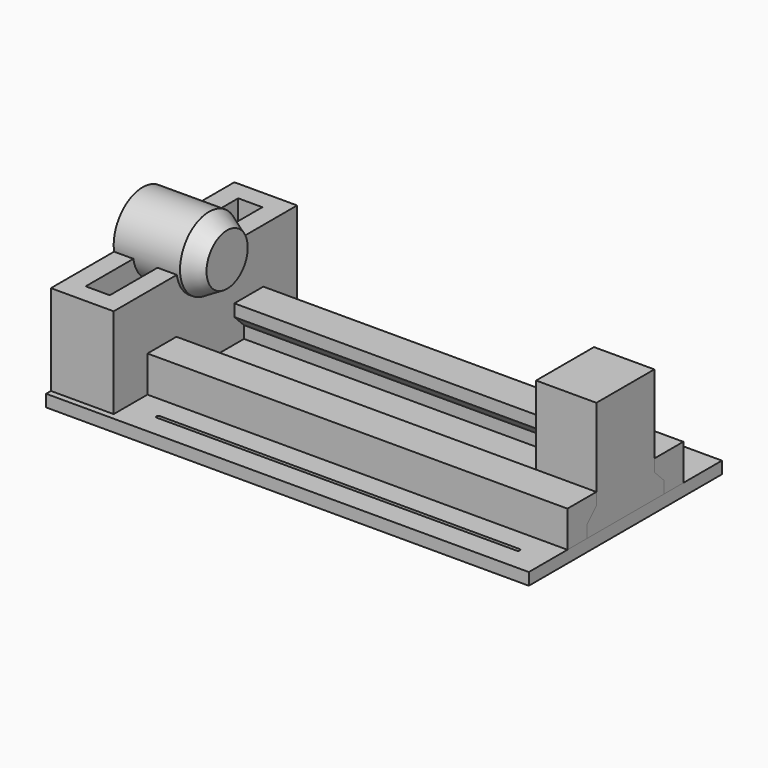
from build123d import *

# Parameters (mm, degrees)
F0_W      = 800
F0_H      = 400
F1_DEPTH  = 20
F2_W      = 40
F2_H      = 32
F3_DEPTH  = 150
F5_DEPTH  = 800.001
F6_R      = 60
F7_DEPTH  = 110
F8_R      = 60
F9_DEPTH  = 30
F9_TAPER  = 30
F11_DEPTH = 696
F14_DEPTH = 100
F17_DEPTH = 20.001


# Not quite as in the source:
# - a pattern or mirror of a feature is missing from the dataset's text; its kind, count and spacing are read off the source's solid


with BuildPart() as f1:
    # F0 (on Top) → F1 (new body)
    with BuildSketch(Plane.XY):
        Rectangle(F0_W, F0_H)
    extrude(amount=F1_DEPTH)

    # F16 (on face) → F17 (cut, through all)
    with BuildSketch(Plane.XY.offset(20)):
        with BuildLine():
            ThreePointArc((-246, -157), (-249, -160), (-246, -163))
            Line((-246, -163), (350, -163))
            ThreePointArc((350, -163), (353, -160), (350, -157))
            Line((350, -157), (-246, -157))
        make_face()
    f17 = extrude(amount=-F17_DEPTH, mode=Mode.SUBTRACT)

    # F17_copies: F17 across plane
    add(f17.mirror(Plane.ZX), mode=Mode.SUBTRACT)


with BuildPart() as f3:
    # F2 (on face) → F3 (new body)
    with BuildSketch(Plane.XY.offset(20)):
        Polygon((-400, 190), (-400, -190), (-368, -190), (-368, -158), (-368, 158), (-368, 190), align=None)
        Polygon((-328, -158), (-328, -190), (-296, -190), (-296, 190), (-328, 190), (-328, 158), align=None)
        with Locations((-348, -174)):
            Rectangle(F2_W, F2_H)
        with Locations((-348, 174)):
            Rectangle(F2_W, F2_H)
    extrude(amount=F3_DEPTH)

    # F4 (on face) → F5 (cut, through all)
    with BuildSketch(Plane(origin=(-400, 0, 0), x_dir=(0, -1, 0), z_dir=(-1, 0, 0))):
        with BuildLine():
            ThreePointArc((59.160797831, 170), (59.7898313673, 174.9824243832), (60, 180))
            ThreePointArc((60, 180), (-5.0175756168, 239.7898313673), (-59.160797831, 170))
            Line((-59.160797831, 170), (59.160797831, 170))
        make_face()
        with BuildLine():
            Line((59.160797831, 170), (-59.160797831, 170))
            ThreePointArc((-59.160797831, 170), (0, 120), (59.160797831, 170))
        make_face()
    extrude(amount=-F5_DEPTH, mode=Mode.SUBTRACT)


with BuildPart() as f7:
    # F6 (on face) → F7 (new body)
    with BuildSketch(Plane(origin=(-400, 0, 0), x_dir=(0, -1, 0), z_dir=(-1, 0, 0))):
        with Locations((0, 180)):
            Circle(F6_R)
    extrude(amount=-F7_DEPTH)

    # F8 (on face) → F9 (join)
    with BuildSketch(Plane.YZ.offset(-290)):
        with Locations((0, 180)):
            Circle(F8_R)
    extrude(amount=F9_DEPTH, taper=F9_TAPER)


with BuildPart() as f11:
    # F10 (on face) → F11 (new body, through all)
    with BuildSketch(Plane.YZ.offset(-296)):
        Polygon((-120, 20), (-80, 20), (-80, 40), (-60, 60), (-60, 80), (-120, 80), align=None)
    extrude(amount=F11_DEPTH)


with BuildPart() as f12_1:
    # F12: instance of F11
    add(f11.part.mirror(Plane.XZ))


with BuildPart() as f14:
    # F13 (on face) → F14 (new body)
    with BuildSketch(Plane.YZ.offset(400)):
        Polygon((-80, 40), (-80, 20), (0, 20), (0, 210), (-60, 210), (-60, 60), align=None)
    extrude(amount=-F14_DEPTH)

    # F15: F14 across face


with BuildPart() as f14_1:
    add(f14.part)
    add(f14.part.mirror(Plane(origin=(350, 0, 115), x_dir=(-1, 0, 0), z_dir=(0, 1, 0))))


solid = Compound([f1.part, f3.part, f7.part, f11.part, f12_1.part, f14_1.part])
